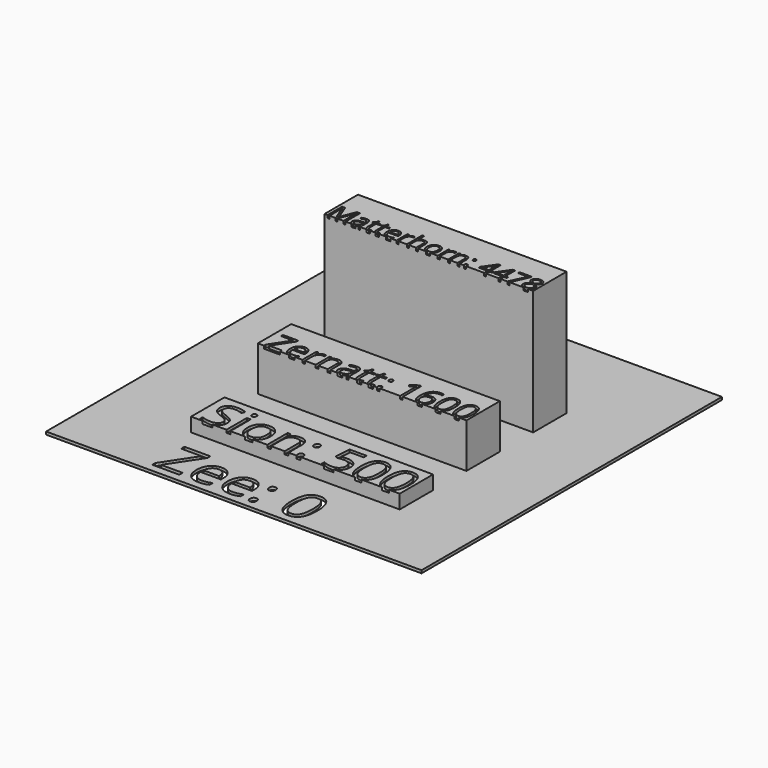
from build123d import *

# Parameters (mm, degrees)
F0_W          = 135
F0_H          = 135
F1_DEPTH      = 1
F2_W          = 74.9999993644
F2_H          = 15
F5_DEPTH      = 5
F3_W          = 75
F3_H          = 15
F6_DEPTH      = 16
F4_W          = 75
F4_H          = 15
F7_DEPTH      = 44.78
F8_TEXT_SIZE  = 9.1249394056
F9_TEXT_SIZE  = 11.7380560418
F10_TEXT_SIZE = 17.1022889191
F11_TEXT_SIZE = 19.8860652745
F12_DEPTH     = 1


# Not quite as in the source:
# - Text() gives the source's letters only with a copy of the font that has no kerning and outlines rounded to 1/6400 em; it was checked with that copy


with BuildPart() as f1:
    # F0 (on Top) → F1 (new body)
    with BuildSketch(Plane.XY):
        with Locations((-1.2300285697, 0.5113658309)):
            Rectangle(F0_W, F0_H)
    extrude(amount=F1_DEPTH)

    # F2 (on face) → F5 (join)
    with BuildSketch(Plane.XY.offset(1)):
        with Locations((0.9075570304, -34.4886341691)):
            Rectangle(F2_W, F2_H)
    extrude(amount=F5_DEPTH)

    # F3 (on face) → F6 (join)
    with BuildSketch(Plane.XY.offset(1)):
        with Locations((0.9075567126, -4.4886341691)):
            Rectangle(F3_W, F3_H)
    extrude(amount=F6_DEPTH)

    # F4 (on face) → F7 (join)
    with BuildSketch(Plane.XY.offset(1)):
        with Locations((0.9075567126, 25.5113658309)):
            Rectangle(F4_W, F4_H)
    extrude(amount=F7_DEPTH)

    # F8 (on face) + F9 (on face) + F10 (on face) + F11 (on face) → F12 (cut)
    with BuildSketch(Plane.XY.offset(45.78)):
        with Locations((-36.4169464136, 18.0113658309)):
            Text('Matterhorn: 4478', F8_TEXT_SIZE, font='Open Sans', text_align=(TextAlign.LEFT, TextAlign.BOTTOM))
    with BuildSketch(Plane.XY.offset(17)):
        with Locations((-34.8837647697, -11.9886341691)):
            Text('Zernatt: 1600', F9_TEXT_SIZE, font='Open Sans', text_align=(TextAlign.LEFT, TextAlign.BOTTOM))
    with BuildSketch(Plane.XY.offset(6)):
        with Locations((-34.7207618126, -41.9886341691)):
            Text('Sion: 500', F10_TEXT_SIZE, font='Open Sans', text_align=(TextAlign.LEFT, TextAlign.BOTTOM))
    with BuildSketch(Plane.XY.offset(1)):
        with Locations((-33.6440578103, -64.1418844461)):
            Text('Zee: 0', F11_TEXT_SIZE, font='Open Sans', text_align=(TextAlign.LEFT, TextAlign.BOTTOM))
    extrude(amount=-F12_DEPTH, mode=Mode.SUBTRACT)


solid = f1.part
